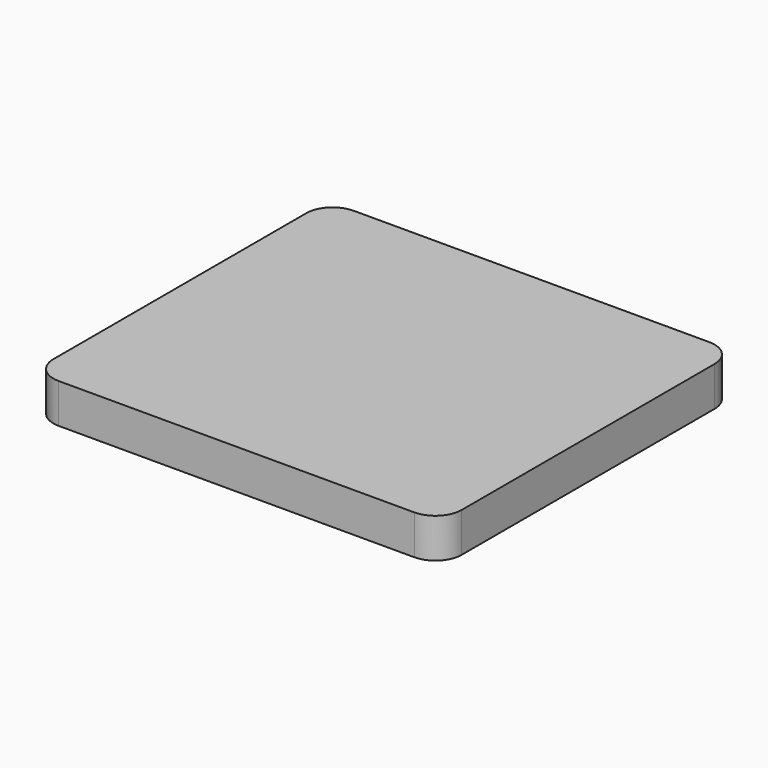
from build123d import *

# Parameters (mm, degrees)
F0_W     = 25
F0_H     = 21
F0_W_2   = 3
F0_H_2   = 6
F0_R     = 3
F0_R_2   = 2.65
F1_DEPTH = 3


with BuildPart() as f1:
    # F0 (on Top) → F1 (new body)
    with BuildSketch(Plane.XY):
        with BuildLine():
            ThreePointArc((15.5, 12), (14.9142135624, 13.4142135624), (13.5, 14))
            Line((13.5, 14), (-13.5, 14))
            ThreePointArc((-13.5, 14), (-14.9142135624, 13.4142135624), (-15.5, 12))
            Line((-15.5, 12), (-15.5, -12))
            ThreePointArc((-15.5, -12), (-14.9142135624, -13.4142135624), (-13.5, -14))
            Line((-13.5, -14), (13.5, -14))
            ThreePointArc((13.5, -14), (14.9142135624, -13.4142135624), (15.5, -12))
            Line((15.5, -12), (15.5, 12))
        make_face()
        Rectangle(F0_W, F0_H, mode=Mode.SUBTRACT)
        Rectangle(F0_W, F0_H)
        with Locations((-7.5, -2.7)):
            Rectangle(F0_W_2, F0_H_2, mode=Mode.SUBTRACT)
        with Locations((7.5, -2.7)):
            Rectangle(F0_W_2, F0_H_2, mode=Mode.SUBTRACT)
        with Locations((-7.5, 5.2)):
            Circle(F0_R, mode=Mode.SUBTRACT)
        with Locations((7.5, 5.2)):
            Circle(F0_R, mode=Mode.SUBTRACT)
        with Locations((7.5, 5.2)):
            Circle(F0_R)
        with Locations((7.5, 5.2)):
            Circle(F0_R_2, mode=Mode.SUBTRACT)
        with Locations((-7.5, 5.2)):
            Circle(F0_R)
        with Locations((-7.5, 5.2)):
            Circle(F0_R_2, mode=Mode.SUBTRACT)
        with Locations((7.5, 5.2)):
            Circle(F0_R_2)
        with Locations((-7.5, 5.2)):
            Circle(F0_R_2)
        with Locations((7.5, -2.7)):
            Rectangle(F0_W_2, F0_H_2)
        with Locations((-7.5, -2.7)):
            Rectangle(F0_W_2, F0_H_2)
    extrude(amount=F1_DEPTH)


solid = f1.part
